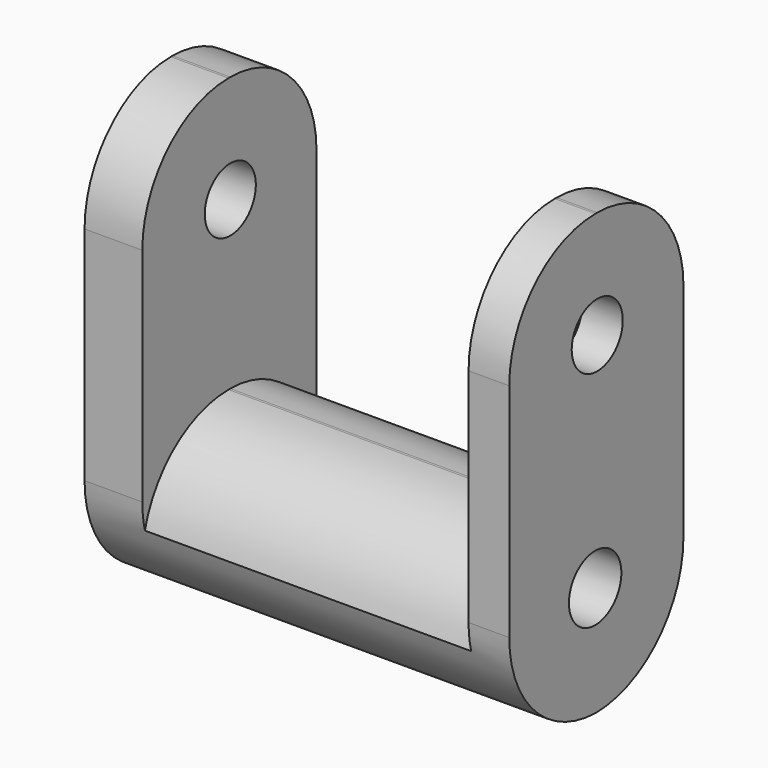
from build123d import *

# Parameters (mm, degrees)
F0_W        = 99.0999639034
F0_H        = 102.6097461581
F1_DEPTH    = 50.8
F2_R        = 25.1416200386
F3_T1_DEPTH = 227.8741153204
F4_R        = 7.4465956944
F4_R_2      = 7.6481080303
F5_DEPTH    = 155.448
F6_W        = 76.1274546385
F6_H        = 70.1917465776
F7_DEPTH    = 112.268
F8_T1_DEPTH = 76.1274546385


# Not quite as in the source:
# - a fillet or chamfer that OpenCascade refuses, or shapes differently, is made with other operations: its cross-section is extruded or revolved along the edge and cut away or added


with BuildPart() as f1:
    # F0 (on Front) → F1 (new body)
    with BuildSketch(Plane.XZ):
        Rectangle(F0_W, F0_H)
    extrude(amount=F1_DEPTH)

    # F2
    f2_edges = [f1.edges().sort_by_distance(p)[0] for p in [
        (0, -50.8, 51.304873),
        (0, 0, 51.304873),
    ]]
    fillet(f2_edges, radius=F2_R)

    # F3: fillet of radius 25.7548302834 on 2 edges, made by hand

    # F3_s2 → F3_t1 (cut)
    with BuildSketch(Plane.YZ.offset(-113.9370576602)):
        with BuildLine():
            ThreePointArc((0, -25.5500427957), (-7.5434151417, -43.7614579374), (-25.7548302834, -51.3048730791))
            Line((-25.7548302834, -51.3048730791), (0, -51.3048730791))
            Line((0, -51.3048730791), (0, -25.5500427957))
        make_face()
        with BuildLine():
            ThreePointArc((-50.8, -25.5500427957), (-43.2565848583, -43.7614579374), (-25.0451697166, -51.3048730791))
            Line((-25.0451697166, -51.3048730791), (-50.8, -51.3048730791))
            Line((-50.8, -51.3048730791), (-50.8, -25.5500427957))
        make_face()
    extrude(amount=F3_T1_DEPTH, mode=Mode.SUBTRACT)

    # F4 (on face) → F5 (cut)
    with BuildSketch(Plane(origin=(-49.5499819517, 0, 0), x_dir=(0, -1, 0), z_dir=(-1, 0, 0))):
        with Locations((25.1416200386, 26.1632530405)):
            Circle(F4_R)
        with Locations((25.7548302834, -25.5500427957)):
            Circle(F4_R_2)
    extrude(amount=-F5_DEPTH, mode=Mode.SUBTRACT)

    # F6 (on Front) → F7 (cut)
    with BuildSketch(Plane.XZ):
        with Locations((1.9891783595, 22.4027493969)):
            Rectangle(F6_W, F6_H)
    extrude(amount=F7_DEPTH, mode=Mode.SUBTRACT)

    # F8: fillet of radius 25.1416200386 on 2 edges, made by hand

    # F8_s2 → F8_t1 (cut)
    with BuildSketch(Plane.YZ.offset(-36.0745489597)):
        with BuildLine():
            ThreePointArc((-50.8, -37.8347439305), (-43.4361899807, -20.0569339112), (-25.6583799614, -12.6931238919))
            Line((-25.6583799614, -12.6931238919), (-50.8, -12.6931238919))
            Line((-50.8, -12.6931238919), (-50.8, -37.8347439305))
        make_face()
        with BuildLine():
            ThreePointArc((0, -37.8347439305), (-7.3638100193, -20.0569339112), (-25.1416200386, -12.6931238919))
            Line((-25.1416200386, -12.6931238919), (0, -12.6931238919))
            Line((0, -12.6931238919), (0, -37.8347439305))
        make_face()
    extrude(amount=F8_T1_DEPTH, mode=Mode.SUBTRACT)


solid = f1.part
